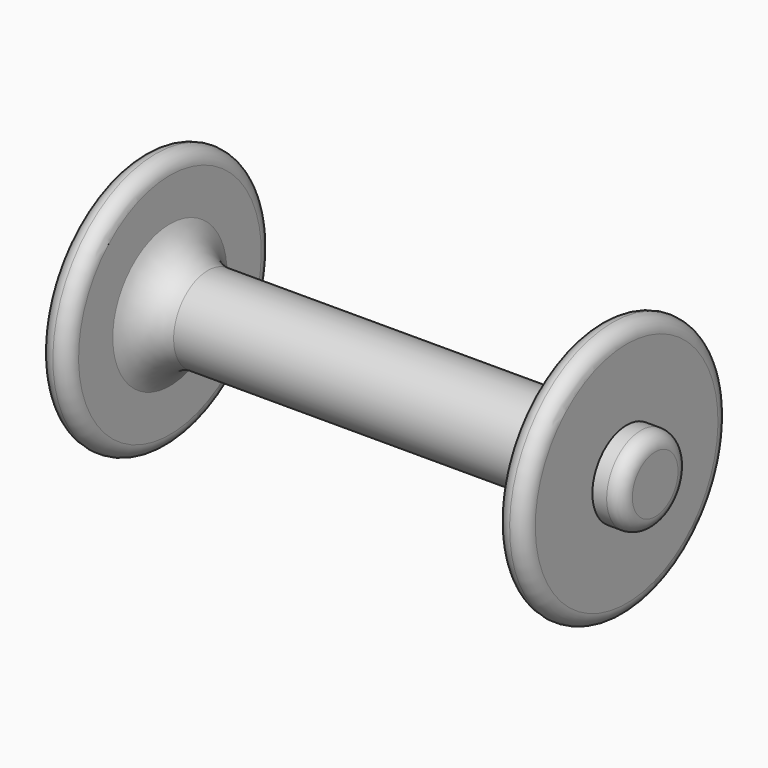
from build123d import *

# Parameters (mm, degrees)
F2_R = 4.99999


# Not quite as in the source:
# - a fillet or chamfer is up to 0.001 mm smaller than in the source, because OpenCascade refuses the exact size


with BuildPart() as f1:
    # F0 (on Front) → F1 (revolve)
    with BuildSketch(Plane.XZ):
        with BuildLine():
            Line((60, 0), (0, 0))
            Line((0, 0), (0, -15))
            Line((0, -15), (95, -15))
            Line((95, -15), (95, 0))
            Line((95, 0), (85, 0))
            Line((85, 0), (85, 30))
            Line((85, 30), (75, 30))
            Line((75, 30), (75, 10))
            Line((75, 10), (75, 0))
            Line((75, 0), (61.6987565648, 0))
            ThreePointArc((61.6987565648, 0), (60.8493782824, -0.0240674236), (60, 0))
        make_face()
        with BuildLine():
            Line((61.6987565648, 0), (60, 0))
            ThreePointArc((60, 0), (60.8493782824, -0.0240674236), (61.6987565648, 0))
        make_face()
        with BuildLine():
            ThreePointArc((75, 10), (69.863256471, 2.9863537681), (61.6987565648, 0))
            Line((61.6987565648, 0), (75, 0))
            Line((75, 0), (75, 10))
        make_face()
    revolve(axis=Axis((47.5, 0, -15), (1, 0, 0)))

    # F2 (radius 5 in the source; OpenCascade refuses exactly that, so slightly less here)
    f2_edges = [f1.edges().sort_by_distance(p)[0] for p in [
        (85, 0, -60),
        (75, 0, -60),
        (95, 0, -30),
    ]]
    fillet(f2_edges, radius=F2_R)

    # F3: F1 across face


with BuildPart() as f1_1:
    add(f1.part)
    add(f1.part.mirror(Plane(origin=(0, 0, -15), x_dir=(0, -1, 0), z_dir=(-1, 0, 0))))


solid = f1_1.part
